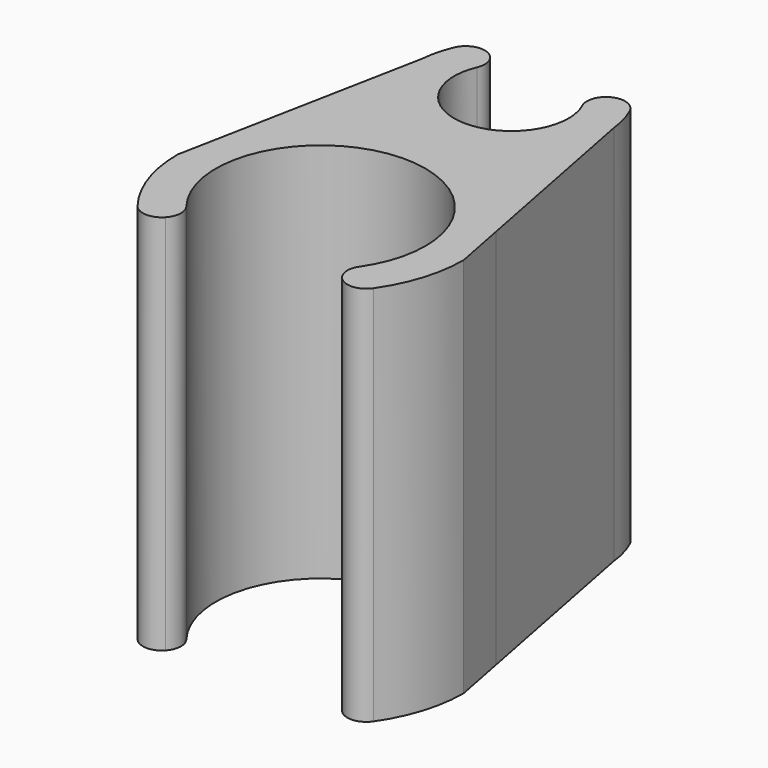
from build123d import *

# Parameters (mm, degrees)
F1_DEPTH = 10
F2_R     = 0.49999


# Not quite as in the source:
# - a fillet or chamfer is up to 0.001 mm smaller than in the source, because OpenCascade refuses the exact size


with BuildPart() as f1:
    # F0 (on Top) → F1 (new body)
    with BuildSketch(Plane.XY):
        with BuildLine():
            Line((-3.4753119677, 1.4087961978), (-3.75, 0))
            ThreePointArc((-3.75, 0), (-3.4444328428, -1.4826943014), (-2.5775293913, -2.723755172))
            Line((-2.5775293913, -2.723755172), (-1.8901882203, -1.9974204595))
            ThreePointArc((-1.8901882203, -1.9974204595), (-1.0873091543, 2.5259174181), (2.75, 0))
            ThreePointArc((2.75, 0), (2.5549370113, -1.0172496587), (1.9974204595, -1.8901882203))
            Line((1.9974204595, -1.8901882203), (2.723755172, -2.5775293913))
            ThreePointArc((2.723755172, -2.5775293913), (3.4840050154, -1.3871586256), (3.75, 0))
            Line((3.75, 0), (3.4774126757, 1.4036028936))
            ThreePointArc((3.4774126757, 1.4036028936), (2.0974972168, 3.1085375059), (0, 3.75))
            ThreePointArc((0, 3.75), (-2.0951747252, 3.1101033537), (-3.4753119677, 1.4087961978))
        make_face()
        with BuildLine():
            Line((-2.4917121164, 6.4533979566), (-3.4753119677, 1.4087961978))
            ThreePointArc((-3.4753119677, 1.4087961978), (-2.0951747252, 3.1101033537), (0, 3.75))
            ThreePointArc((0, 3.75), (-1.8382729519, 4.5556704706), (-2.4917121164, 6.4533979566))
        make_face()
        with BuildLine():
            ThreePointArc((2.5, 6.25), (1.767766953, 4.482233047), (0, 3.75))
            ThreePointArc((0, 3.75), (2.0974972168, 3.1085375059), (3.4774126757, 1.4036028936))
            Line((3.4774126757, 1.4036028936), (2.4872564888, 6.5021014854))
            ThreePointArc((2.4872564888, 6.5021014854), (2.4968120896, 6.3762116833), (2.5, 6.25))
        make_face()
        with BuildLine():
            ThreePointArc((-2.4917121164, 6.4533979566), (-1.8382729519, 4.5556704706), (0, 3.75))
            ThreePointArc((0, 3.75), (1.767766953, 4.482233047), (2.5, 6.25))
            ThreePointArc((2.5, 6.25), (2.4968120896, 6.3762116833), (2.4872564888, 6.5021014854))
            ThreePointArc((2.4872564888, 6.5021014854), (2.3111850264, 7.2031126763), (1.9419288742, 7.8244561752))
            Line((1.9419288742, 7.8244561752), (1.1651573245, 7.1946737051))
            ThreePointArc((1.1651573245, 7.1946737051), (1.4138132809, 6.7511307281), (1.5, 6.25))
            ThreePointArc((1.5, 6.25), (-0.4879304654, 4.831576981), (-1.1825651479, 7.1727890718))
            Line((-1.1825651479, 7.1727890718), (-1.9709419132, 7.7879817863))
            ThreePointArc((-1.9709419132, 7.7879817863), (-2.3289694602, 7.1587910945), (-2.4917121164, 6.4533979566))
        make_face()
    extrude(amount=F1_DEPTH)

    # F2 (radius 0.5 in the source; OpenCascade refuses exactly that, so slightly less here)
    f2_edges = [f1.edges().sort_by_distance(p)[0] for p in [
        (-1.182565, 7.172789, 5),
        (1.165157, 7.194674, 5),
        (-1.890188, -1.99742, 5),
        (1.99742, -1.890188, 5),
        (-1.970942, 7.787982, 5),
        (1.941929, 7.824456, 5),
        (2.723755, -2.577529, 5),
        (-2.577529, -2.723755, 5),
    ]]
    fillet(f2_edges, radius=F2_R)


solid = f1.part
